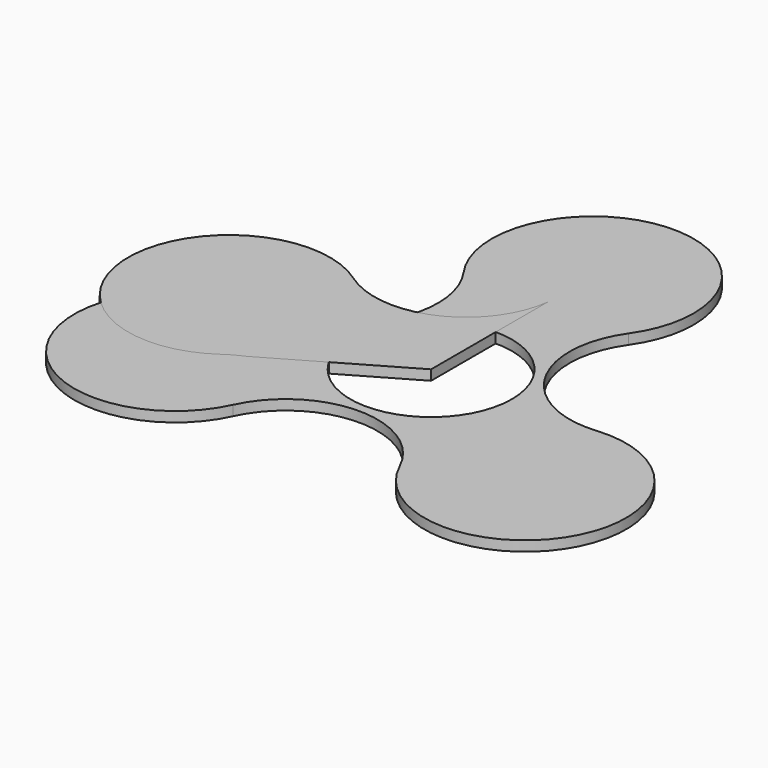
from build123d import *

# Parameters (mm, degrees)
F0_R     = 100
F1_DEPTH = 12.5
F3_DEPTH = 12.5
F5_ANGLE = 90


# Not quite as in the source:
# - a feature names something its author has since deleted; it is built from what else it names


with BuildPart() as f1:
    # F0 (on Top) → F1 (new body)
    with BuildSketch(Plane.XY):
        with BuildLine():
            ThreePointArc((205.1583347086, -0.5161756393), (96.5749958013, 55.7575998229), (102.1321461379, 177.9304174754))
            ThreePointArc((102.1321461379, 177.9304174754), (0, 375), (-102.1321461379, 177.9304174754))
            ThreePointArc((-102.1321461379, 177.9304174754), (-96.5749958013, 55.7575998229), (-205.1583347086, -0.5161756393))
            ThreePointArc((-205.1583347086, -0.5161756393), (-324.7595264192, -187.5), (-103.0261885707, -177.4142418361))
            ThreePointArc((-103.0261885707, -177.4142418361), (0, -111.5151996458), (103.0261885707, -177.4142418361))
            ThreePointArc((103.0261885707, -177.4142418361), (324.7595264192, -187.5), (205.1583347086, -0.5161756393))
        make_face()
        Circle(F0_R, mode=Mode.SUBTRACT)
    extrude(amount=F1_DEPTH)


with BuildPart() as f3:
    # F2 (on Top) → F3 (new body)
    with BuildSketch(Plane.XY):
        with BuildLine():
            ThreePointArc((179.9376090198, 0), (90.877396005, 67.0323311206), (102.1321461379, 177.9304174754))
            ThreePointArc((102.1321461379, 177.9304174754), (0, 375), (-102.1321461379, 177.9304174754))
            ThreePointArc((-102.1321461379, 177.9304174754), (-95.4345073685, 167.2194957508), (-89.9688045099, 155.8305405074))
            Line((-89.9688045099, 155.8305405074), (0, 0))
            Line((0, 0), (179.9376090198, 0))
        make_face()
    extrude(amount=F3_DEPTH)


with BuildPart() as f3_1:
    # F5: moved
    add(f3.part.rotate(Axis((0, 0, 34.5875732601), (0, 0, 1)), F5_ANGLE))


solid = Compound([f1.part, f3_1.part])
